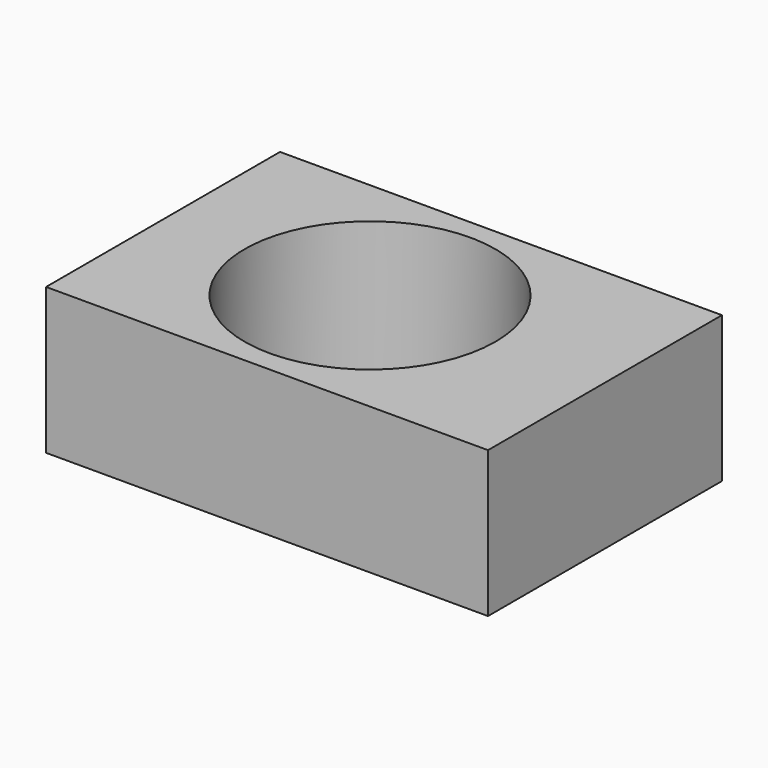
from build123d import *

# Parameters (mm, degrees)
F0_W     = 76.8432989717
F0_H     = 50.8419405669
F0_R     = 21.8075174345
F1_DEPTH = 25.4
F2_DEPTH = 25.4


# Not quite as in the source:
# - the program builds the solid bodies; features that only make, move or delete a surface that nothing else refers to are left out


with BuildPart() as f1:
    # F0 (on Top) → F1 (new body)
    with BuildSketch(Plane.XY):
        with Locations((2.5134049356, -0.1019602641)):
            Rectangle(F0_W, F0_H)
        Circle(F0_R, mode=Mode.SUBTRACT)
    extrude(amount=F1_DEPTH)


with BuildPart() as f2:
    # F0 (on Top) → F2 (new body)
    with BuildSketch(Plane.XY):
        with Locations((2.5134049356, -0.1019602641)):
            Rectangle(F0_W, F0_H)
        Circle(F0_R, mode=Mode.SUBTRACT)
    extrude(amount=F2_DEPTH)


solid = Compound([f1.part, f2.part])
